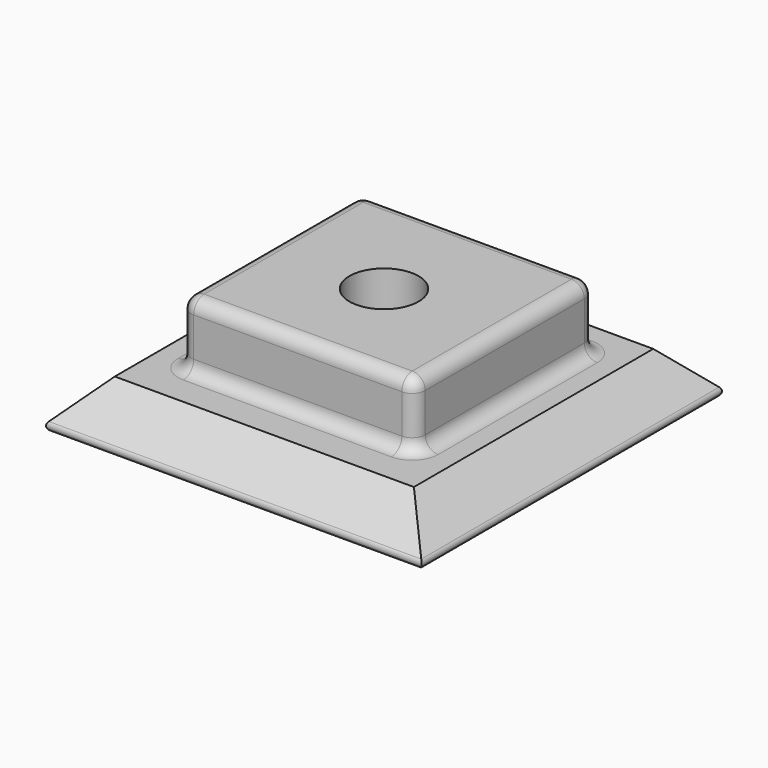
from build123d import *

# Parameters (mm, degrees)
F0_W      = 38.1
F0_H      = 38.1
F1_DEPTH  = 4.445
F4_DEPTH  = 38.101
F5_DEPTH  = 38.101
F6_R      = 0.508
F7_W      = 22.86
F7_H      = 21.9536569705
F8_DEPTH  = 6.35
F9_R      = 3.3734375
F10_DEPTH = 10.7965917968
F11_R     = 9.525
F12_DEPTH = 3.175
F13_R     = 1.27


with BuildPart() as f1:
    # F0 (on Top) → F1 (new body)
    with BuildSketch(Plane.XY):
        Rectangle(F0_W, F0_H)
    extrude(amount=F1_DEPTH)

    # F2 (on face) → F4 (cut, through all)
    with BuildSketch(Plane.XZ.offset(19.05)):
        Polygon((-19.05, 4.445), (-19.05, 0), (-14.605, 4.445), align=None)
        Polygon((14.605, 4.445), (19.05, 0), (19.05, 4.445), align=None)
    extrude(amount=-F4_DEPTH, mode=Mode.SUBTRACT)

    # F3 (on face) → F5 (cut, through all)
    with BuildSketch(Plane(origin=(-19.05, 0, 0), x_dir=(0, -1, 0), z_dir=(-1, 0, 0))):
        Polygon((-19.05, 4.445), (-19.05, 0), (-14.605, 4.445), align=None)
        Polygon((14.605, 4.445), (19.05, 0), (19.05, 4.445), align=None)
    extrude(amount=-F5_DEPTH, mode=Mode.SUBTRACT)

    # F6
    f6_edges = [f1.edges().sort_by_distance(p)[0] for p in [
        (19.05, 0, 0),
        (0, -19.05, 0),
        (-19.05, 0, 0),
        (0, 19.05, 0),
    ]]
    fillet(f6_edges, radius=F6_R)

    # F7 (on face) → F8 (join)
    with BuildSketch(Plane.XY.offset(4.445)):
        with Locations((0, 0.4531715147)):
            Rectangle(F7_W, F7_H)
    extrude(amount=F8_DEPTH)

    # F9 (on face) → F10 (cut, through all)
    with BuildSketch(Plane.XY.offset(10.795)):
        Circle(F9_R)
    extrude(amount=-F10_DEPTH, mode=Mode.SUBTRACT)

    # F11 (on face) → F12 (cut)
    with BuildSketch(Plane(origin=(0, 0, 0), x_dir=(1, 0, 0), z_dir=(0, 0, -1))):
        Circle(F11_R)
    extrude(amount=-F12_DEPTH, mode=Mode.SUBTRACT)

    # F13
    f13_edges = [f1.edges().sort_by_distance(p)[0] for p in [
        (-11.43, 0.453172, 4.445),
        (0, -10.523657, 4.445),
        (-11.43, -10.523657, 7.62),
        (-11.43, 11.43, 7.62),
        (11.43, 11.43, 7.62),
        (11.43, -10.523657, 7.62),
        (0, 11.43, 10.795),
        (11.43, 0.453172, 10.795),
        (0, -10.523657, 10.795),
        (-18.18279, 0, 0.86721),
        (-11.43, 0.453172, 10.795),
        (11.43, 0.453172, 4.445),
        (0, 11.43, 4.445),
    ]]
    fillet(f13_edges, radius=F13_R)


solid = f1.part
